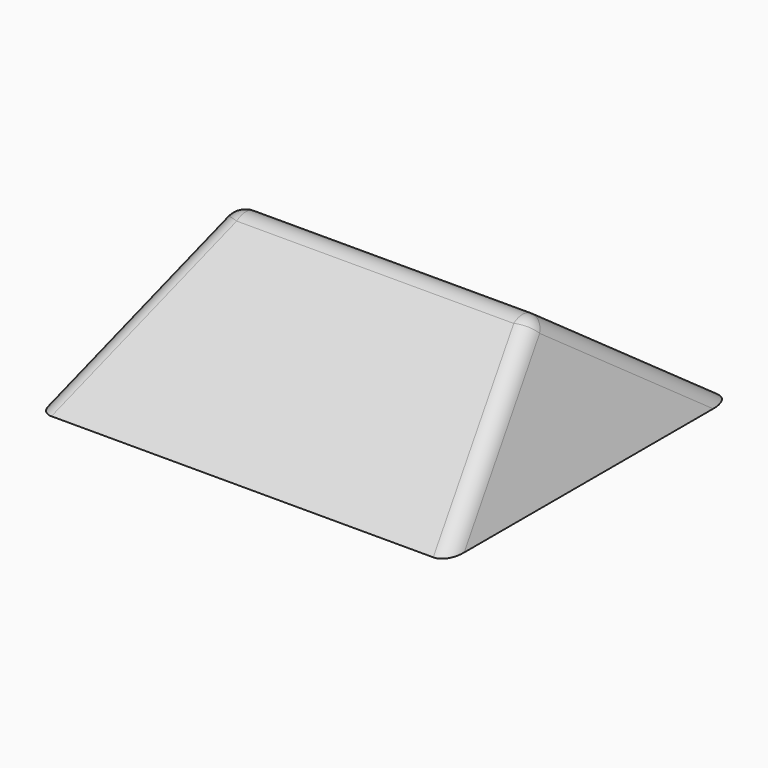
from build123d import *

# Parameters (mm, degrees)
F0_W      = 63.5
F0_H      = 44.45
F0_W_2    = 50.292
F0_H_2    = 31.242
F1_DEPTH  = 1.5875
F2_W      = 50.292
F2_H      = 31.242
F2_W_2    = 47.117
F2_H_2    = 28.067
F3_DEPTH  = 6.35
F5_DEPTH  = 34.925
F7_DEPTH  = 38.1
F9_DEPTH  = 38.1
F11_DEPTH = 38.1
F12_R     = 3.175
F14_DEPTH = 50.292
F15_W     = 28.575
F15_H     = 4.7625
F16_DEPTH = 50.292


with BuildPart() as f1:
    # F0 (on Top) → F1 (new body)
    with BuildSketch(Plane.XY):
        Rectangle(F0_W, F0_H)
        Rectangle(F0_W_2, F0_H_2, mode=Mode.SUBTRACT)
    extrude(amount=F1_DEPTH)

    # F2 (on face) → F3 (join)
    with BuildSketch(Plane.XY.offset(1.5875)):
        Rectangle(F2_W, F2_H)
        Rectangle(F2_W_2, F2_H_2, mode=Mode.SUBTRACT)
    extrude(amount=-F3_DEPTH)

    # F4 (on Right) → F5 (join, symmetric)
    with BuildSketch(Plane.YZ):
        Polygon((-15.6114658074, 4.507067833), (0, 15.1461502537), (15.6114658074, 4.507067833), (15.6114658074, 0), (22.225, 0), (29.2133475819, -4.7625), (32.3883475819, -4.7625), (0, 17.3098860042), (-32.3883475819, -4.7625), (-29.2133475819, -4.7625), (-22.225, 0), (-15.6114658074, 0), align=None)
    extrude(amount=F5_DEPTH, both=True)

    # F6 (on Front) → F7 (cut, symmetric)
    with BuildSketch(Plane.XZ):
        Polygon((-34.925, -4.7625), (-25.4, 17.3098860042), (-34.925, 17.3098860042), align=None)
        Polygon((34.925, -4.7625), (34.925, 17.3098860042), (25.4, 17.3098860042), align=None)
    extrude(amount=F7_DEPTH, both=True, mode=Mode.SUBTRACT)

    # F8 (on Front) → F9 (join, symmetric)
    with BuildSketch(Plane.XZ):
        Polygon((-23.8125, 17.3098860042), (-25.4, 17.3098860042), (-34.925, -4.7625), (-33.3375, -4.7625), align=None)
        Polygon((34.925, -4.7625), (25.4, 17.3098860042), (23.8125, 17.3098860042), (33.3375, -4.7625), align=None)
    extrude(amount=F9_DEPTH, both=True)

    # F10 (on Right) → F11 (cut, symmetric)
    with BuildSketch(Plane.YZ):
        Polygon((-30.21584, -4.7625), (0, 17.3098860042), (-38.1, 17.3098860042), (-38.1, -4.7625), align=None)
        Polygon((38.1, 17.3098860042), (0, 17.3098860042), (30.21584, -4.7625), (38.1, -4.7625), align=None)
    extrude(amount=F11_DEPTH, both=True, mode=Mode.SUBTRACT)

    # F12
    f12_edges = [f1.edges().sort_by_distance(p)[0] for p in [
        (30.1625, -15.10792, 6.273693),
        (30.1625, 15.10792, 6.273693),
        (0, 0, 17.309886),
        (-30.1625, -15.10792, 6.273693),
        (-30.1625, 15.10792, 6.273693),
    ]]
    fillet(f12_edges, radius=F12_R)

    # F13 (on face) → F14 (join, through all)
    with BuildSketch(Plane.YZ.offset(25.146)):
        with BuildLine():
            Line((-15.621, -4.7625), (-15.621, -2.7305))
            ThreePointArc((-15.621, -2.7305), (-16.637, -3.7465), (-15.621, -4.7625))
        make_face()
        with BuildLine():
            ThreePointArc((15.621, -4.7625), (16.637, -3.7465), (15.621, -2.7305))
            Line((15.621, -2.7305), (15.621, -4.7625))
        make_face()
    extrude(amount=-F14_DEPTH)

    # F15 (on face) → F16 (cut, through all)
    with BuildSketch(Plane.YZ.offset(25.146)):
        with Locations((0, -2.38125)):
            Rectangle(F15_W, F15_H)
    extrude(amount=-F16_DEPTH, mode=Mode.SUBTRACT)


solid = f1.part
